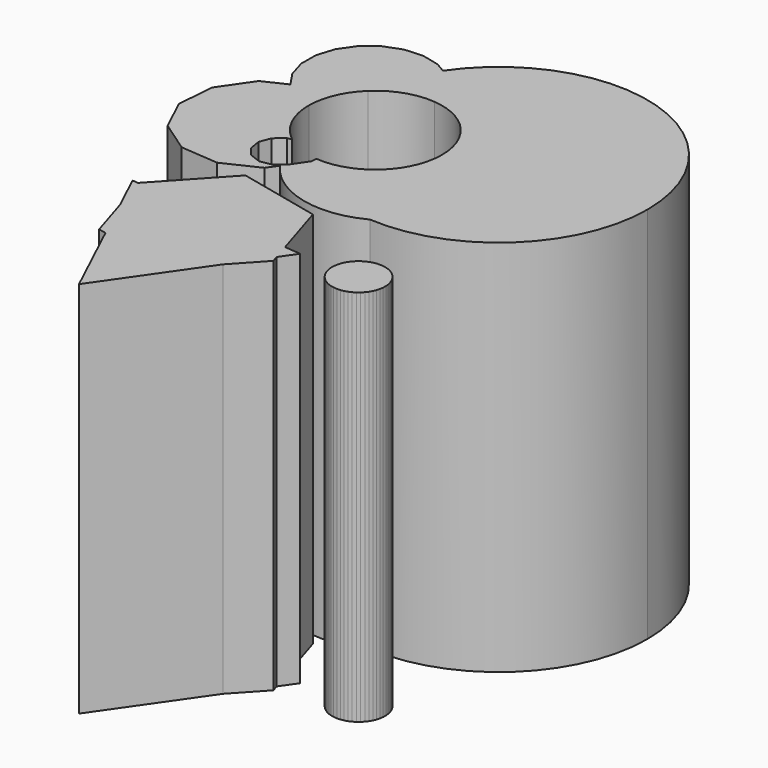
from build123d import *

# Parameters (mm, degrees)
F1_DEPTH = 254


with BuildPart() as f1:
    # F0 (on Top) → F1 (new body)
    with BuildSketch(Plane.XY):
        with BuildLine():
            ThreePointArc((-96.3984984512, -11.1761820134), (-88.2280728921, -24.8950502892), (-85.3843353303, -40.607349843))
            ThreePointArc((-85.3843353303, -40.607349843), (-99.9057947256, -73.6389869304), (-134.0622763632, -85.2706933306))
            Line((-134.0622763632, -85.2706933306), (-134.3795441197, -89.2403272416))
            Line((-134.3795441197, -89.2403272416), (-135.1082130036, -90.2977937911))
            ThreePointArc((-135.1082130036, -90.2977937911), (-105.053863362, -112.2168709289), (-69.0635469875, -121.6193707149))
            ThreePointArc((-69.0635469875, -121.6193707149), (-46.0665525367, -100.0654924355), (-37.5807690897, -69.7105438777))
            ThreePointArc((-37.5807690897, -69.7105438777), (-54.8253518386, -28.2201931739), (-96.3984984512, -11.1761820134))
        make_face()
        with BuildLine():
            ThreePointArc((-126.2687263791, 4.047665135), (-109.8568709833, -0.6667908851), (-96.3984984512, -11.1761820134))
            ThreePointArc((-96.3984984512, -11.1761820134), (-54.8253518386, -28.2201931739), (-37.5807690897, -69.7105438777))
            ThreePointArc((-37.5807690897, -69.7105438777), (-46.0665525367, -100.0654924355), (-69.0635469875, -121.6193707149))
            ThreePointArc((-69.0635469875, -121.6193707149), (5.927575035, -94.9642404509), (37.6343625868, -21.965309125))
            ThreePointArc((37.6343625868, -21.965309125), (-32.7893321574, 73.4771630738), (-144.7578393906, 34.3387462838))
            Line((-144.7578393906, 34.3387462838), (-140.9298784761, 32.0858849303))
            Line((-140.9298784761, 32.0858849303), (-132.6287708701, 22.9883655039))
            Line((-132.6287708701, 22.9883655039), (-127.3779991091, 11.8482289198))
            Line((-127.3779991091, 11.8482289198), (-126.2687263791, 4.047665135))
        make_face()
        with BuildLine():
            ThreePointArc((-161.1854910333, -8.1982733406), (-145.0495253406, 1.695293838), (-126.2687263791, 4.047665135))
            Line((-126.2687263791, 4.047665135), (-127.3779991091, 11.8482289198))
            Line((-127.3779991091, 11.8482289198), (-132.6287708701, 22.9883655039))
            Line((-132.6287708701, 22.9883655039), (-140.9298784761, 32.0858849303))
            Line((-140.9298784761, 32.0858849303), (-144.7578393906, 34.3387462838))
            ThreePointArc((-144.7578393906, 34.3387462838), (-155.431440726, 14.0201933708), (-161.1854910333, -8.1982733406))
        make_face()
        with BuildLine():
            ThreePointArc((-172.4459379951, -25.5731395571), (-167.8325516116, -16.226706255), (-161.1854910333, -8.1982733406))
            ThreePointArc((-161.1854910333, -8.1982733406), (-155.431440726, 14.0201933708), (-144.7578393906, 34.3387462838))
            Line((-144.7578393906, 34.3387462838), (-151.5437320876, 38.332432674))
            Line((-151.5437320876, 38.332432674), (-163.527244233, 41.1729755555))
            Line((-163.527244233, 41.1729755555), (-175.8156272694, 40.3551188743))
            Line((-175.8156272694, 40.3551188743), (-187.3170044373, 35.9515327856))
            Line((-187.3170044373, 35.9515327856), (-197.0094279025, 28.3534952382))
            Line((-197.0094279025, 28.3534952382), (-204.0316833055, 18.2361252116))
            Line((-204.0316833055, 18.2361252116), (-207.7598124371, 6.498395432))
            Line((-207.7598124371, 6.498395432), (-207.8625546634, -5.8167452994))
            Line((-207.8625546634, -5.8167452994), (-204.3307808867, -17.6150426846))
            Line((-204.3307808867, -17.6150426846), (-197.4853327932, -27.8376708531))
            Line((-197.4853327932, -27.8376708531), (-189.8049237905, -24.1857455048))
            Line((-189.8049237905, -24.1857455048), (-172.4459379951, -25.5731395571))
        make_face()
        with BuildLine():
            ThreePointArc((-144.0610363204, -103.290404551), (-110.0124554075, -126.5720842598), (-69.0635469875, -121.6193707149))
            ThreePointArc((-69.0635469875, -121.6193707149), (-105.053863362, -112.2168709289), (-135.1082130036, -90.2977937911))
            Line((-135.1082130036, -90.2977937911), (-141.6257801704, -99.7562864145))
            Line((-141.6257801704, -99.7562864145), (-144.0610363204, -103.290404551))
        make_face()
        with BuildLine():
            ThreePointArc((-175.0412102144, -40.3222661109), (-174.3638249729, -32.8385628221), (-172.4459379951, -25.5731395571))
            Line((-172.4459379951, -25.5731395571), (-189.8049237905, -24.1857455048))
            Line((-189.8049237905, -24.1857455048), (-197.4853327932, -27.8376708531))
            Line((-197.4853327932, -27.8376708531), (-197.4783047059, -27.848166225))
            Line((-197.4783047059, -27.848166225), (-187.9139987013, -35.6068579866))
            Line((-187.9139987013, -35.6068579866), (-176.4876934338, -40.2017241579))
            Line((-176.4876934338, -40.2017241579), (-175.0412102144, -40.3222661109))
        make_face()
        with BuildLine():
            Line((-148.8720162211, -110.2722455874), (-144.0610363204, -103.290404551))
            ThreePointArc((-144.0610363204, -103.290404551), (-144.3963145668, -102.8065353405), (-144.7267097272, -102.319318804))
            Line((-144.7267097272, -102.319318804), (-147.8276392839, -104.8823511934))
            Line((-147.8276392839, -104.8823511934), (-155.7616392164, -106.2207239567))
            Line((-155.7616392164, -106.2207239567), (-163.3018710931, -103.4127888031))
            Line((-163.3018710931, -103.4127888031), (-168.4279358721, -97.2109296896))
            Line((-168.4279358721, -97.2109296896), (-169.7663086353, -89.2769297572))
            Line((-169.7663086353, -89.2769297572), (-166.9583734818, -81.7366978804))
            Line((-166.9583734818, -81.7366978804), (-160.7565143683, -76.6106331015))
            Line((-160.7565143683, -76.6106331015), (-157.6211982017, -76.0817420254))
            ThreePointArc((-157.6211982017, -76.0817420254), (-170.5145086023, -60.2398754557), (-175.0412102144, -40.3222661109))
            Line((-175.0412102144, -40.3222661109), (-176.4876934338, -40.2017241579))
            Line((-176.4876934338, -40.2017241579), (-187.9139987013, -35.6068579866))
            Line((-187.9139987013, -35.6068579866), (-197.4783047059, -27.848166225))
            Line((-197.4783047059, -27.848166225), (-197.4853327932, -27.8376708531))
            Line((-197.4853327932, -27.8376708531), (-212.8717319669, -35.1536850318))
            Line((-212.8717319669, -35.1536850318), (-227.3642040683, -56.1856033777))
            Line((-227.3642040683, -56.1856033777), (-229.3990938989, -81.6460150062))
            Line((-229.3990938989, -81.6460150062), (-218.4311543718, -104.7128231825))
            Line((-218.4311543718, -104.7128231825), (-197.399236026, -119.2052952839))
            Line((-197.399236026, -119.2052952839), (-171.9388243975, -121.2401851145))
            Line((-171.9388243975, -121.2401851145), (-148.8720162211, -110.2722455874))
        make_face()
        with BuildLine():
            ThreePointArc((-144.7267097272, -102.319318804), (-144.3963145668, -102.8065353405), (-144.0610363204, -103.290404551))
            Line((-144.0610363204, -103.290404551), (-141.6257801704, -99.7562864145))
            Line((-141.6257801704, -99.7562864145), (-144.7267097272, -102.319318804))
        make_face()
    extrude(amount=F1_DEPTH)


with BuildPart() as f1b:
    # F0 (on Top) → F1, piece 2 (new body)
    with BuildSketch(Plane.XY):
        Polygon((-80.6372836352, -185.3906590886), (-73.2946771071, -174.8100775029), (-84.2030009787, -173.9018466033), align=None)
        Polygon((-79.2373413166, -189.9013011951), (-80.6372836352, -185.3906590886), (-97.3969621498, -209.5410946584), align=None)
        Polygon((-97.3969621498, -209.5410946584), (-80.6372836352, -185.3906590886), (-84.2030009787, -173.9018466033), (-189.7292425711, -165.115694444), (-181.8896663365, -190.3749656225), (-167.8424976004, -220.172014917), (-117.7198875587, -231.5205215015), align=None)
        Polygon((-189.7292425711, -165.115694444), (-84.2030009787, -173.9018466033), (-96.0393702666, -135.764828394), (-151.3239454586, -123.2475758992), (-189.8064917008, -164.8667962055), align=None)
        Polygon((-142.3301619603, -274.289135382), (-97.3969621498, -209.5410946584), (-117.7198875587, -231.5205215015), (-167.8424976004, -220.172014917), align=None)
        Polygon((-181.8896663365, -190.3749656225), (-189.7292425711, -165.115694444), (-193.9638108015, -164.763122797), align=None)
        Polygon((-167.8424976004, -220.172014917), (-181.8896663365, -190.3749656225), (-173.0044627508, -219.0032690067), align=None)
    extrude(amount=F1_DEPTH)


with BuildPart() as f1c:
    # F0 (on Top) → F1, piece 3 (new body)
    with BuildSketch(Plane.XY):
        Polygon((-30.4232937559, -158.5347692393), (-32.6511874007, -158.3492740272), (-34.8847621535, -158.4444706149), (-37.0887932061, -158.8188576952), (-39.2285216721, -159.4665309603), (-41.2702027554, -160.3772762158), (-43.1816379258, -161.536730465), (-44.9326827087, -162.9266084218), (-46.4957220818, -164.5249908806), (-47.8461059807, -166.306670395), (-48.9625380444, -168.243548815), (-49.8274114725, -170.3050804106), (-50.4270866943, -172.4587535973), (-50.7521064733, -174.6706036622), (-50.7973450534, -176.9057484086), (-50.5620889954, -179.1289382686), (-50.0500484276, -181.3051122101), (-49.2692985357, -183.3999506699), (-48.232152212, -185.3804167943), (-46.9549658735, -187.2152774493), (-45.4578815117, -188.8755957863), (-43.7645090414, -190.3351875933), (-41.9015539579, -191.5710342356), (-39.8983961758, -192.5636456735), (-37.7866266899, -193.2973678315), (-35.5995493666, -193.7606294729), (-33.3716557217, -193.9461246849), (-31.138080969, -193.8509280972), (-28.9340499164, -193.4765410169), (-26.7943214504, -192.8288677519), (-24.7526403671, -191.9181224964), (-22.8412051967, -190.7586682471), (-21.0901604138, -189.3687902903), (-19.5271210406, -187.7704078316), (-18.1767371418, -185.9887283171), (-17.0603050781, -184.0518498972), (-16.19543165, -181.9903183015), (-15.5957564282, -179.8366451149), (-15.2707366492, -177.62479505), (-15.225498069, -175.3896503035), (-15.4607541271, -173.1664604435), (-15.9727946949, -170.9902865021), (-16.7535445868, -168.8954480422), (-17.7906909105, -166.9149819179), (-19.067877249, -165.0801212629), (-20.5649616108, -163.4198029259), (-22.2583340811, -161.9602111188), (-24.1212891646, -160.7243644765), (-26.1244469467, -159.7317530387), (-28.2362164326, -158.9980308807), align=None)
    extrude(amount=F1_DEPTH)


solid = Compound([f1.part, f1b.part, f1c.part])
